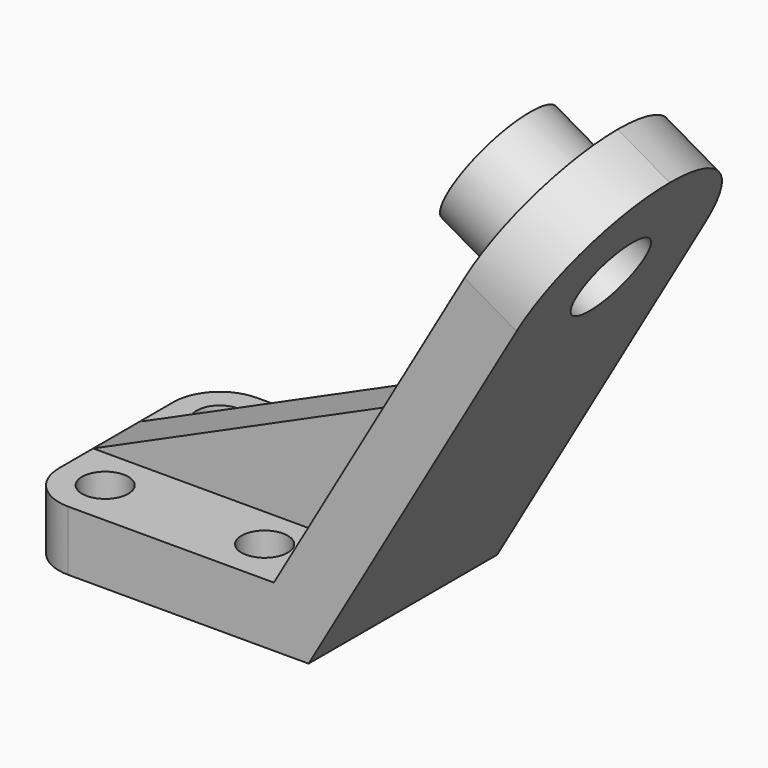
from build123d import *

# Parameters (mm, degrees)
F1_DEPTH  = 102
F2_R      = 50.99999
F3_R      = 27
F3_R_2    = 18.5
F4_DEPTH  = 30
F5_R      = 18.5
F6_DEPTH  = 30
F7_R      = 10
F8_DEPTH  = 30
F11_DEPTH = 12.5
F12_R     = 20


# Not quite as in the source:
# - a fillet or chamfer is up to 0.001 mm smaller than in the source, because OpenCascade refuses the exact size


with BuildPart() as f1:
    # F0 (on Front) → F1 (new body)
    with BuildSketch(Plane.XZ):
        Polygon((-36.2992759747, -102.7012261555), (-145.2992759747, -102.7012261555), (-145.2992759747, -128.7012261555), (-21.2881689757, -128.7012261555), (94.2118310243, 71.3506421187), (71.6951705259, 84.3506421187), align=None)
    extrude(amount=F1_DEPTH)

    # F2 (radius 51 in the source; OpenCascade refuses exactly that, so slightly less here)
    f2_edges = [f1.edges().sort_by_distance(p)[0] for p in [
        (82.953501, 0, 77.850642),
        (82.953501, -102, 77.850642),
    ]]
    fillet(f2_edges, radius=F2_R)

    # F3 (on face) → F4 (join)
    with BuildSketch(Plane(origin=(17.2464784442, 0, -9.9572589724), x_dir=(0, -1, 0), z_dir=(-0.8660254038, 0, 0.5))):
        with Locations((51, 57.8973841632)):
            Circle(F3_R)
        with Locations((51, 57.8973841632)):
            Circle(F3_R_2, mode=Mode.SUBTRACT)
    extrude(amount=F4_DEPTH)

    # F5 (on face) → F6 (cut)
    with BuildSketch(Plane(origin=(17.2464784442, 0, -9.9572589724), x_dir=(0, -1, 0), z_dir=(-0.8660254038, 0, 0.5))):
        with Locations((51, 57.8973841632)):
            Circle(F5_R)
    extrude(amount=-F6_DEPTH, mode=Mode.SUBTRACT)

    # F7 (on face) → F8 (cut)
    with BuildSketch(Plane.XY.offset(-102.7012261555)):
        with Locations((-125.2992759747, -20)):
            Circle(F7_R)
        with Locations((-125.2992759747, -82)):
            Circle(F7_R)
        with Locations((-56.2992759747, -20)):
            Circle(F7_R)
        with Locations((-56.2992759747, -82)):
            Circle(F7_R)
    extrude(amount=-F8_DEPTH, mode=Mode.SUBTRACT)

    # F10 (on offset) → F11 (join, symmetric)
    with BuildSketch(Plane.XZ.offset(51)):
        Polygon((-35.6261391794, -102.7012261555), (1.8678903299, -36.5937549351), (-145.2992759747, -102.7012261555), align=None)
    extrude(amount=F11_DEPTH, both=True)

    # F12
    f12_edges = [f1.edges().sort_by_distance(p)[0] for p in [
        (-145.299276, 0, -115.701226),
        (-145.299276, -102, -115.701226),
    ]]
    fillet(f12_edges, radius=F12_R)


solid = f1.part
